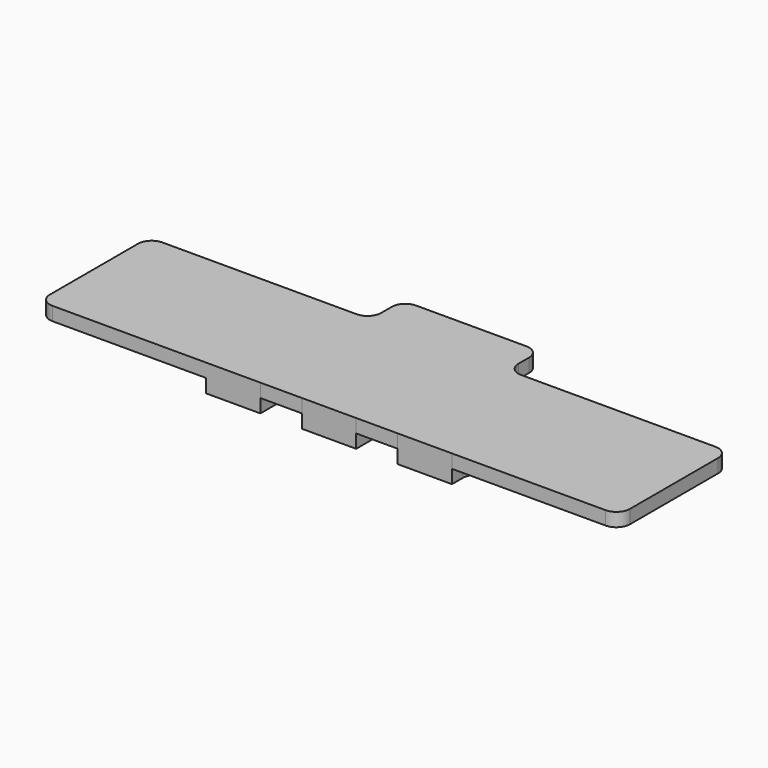
from build123d import *

# Parameters (mm, degrees)
F1_DEPTH = 0.75
F2_DEPTH = 0.75


# Not quite as in the source:
# - ends of sketch curves that miss each other by under 0.0002 mm in the source are joined


with BuildPart() as f1:
    # F0 (on Top) → F1 (new body)
    with BuildSketch(Plane.XY):
        with BuildLine():
            Line((-4.3542903055, 3.0103204122), (-15.1042902548, 3.0103204122))
            ThreePointArc((-15.1042902548, 3.0103204122), (-15.634620706, 2.7906503467), (-15.8542907714, 2.2603198956))
            Line((-15.8542907714, 2.2603198956), (-15.8542907714, -3.8396952234))
            ThreePointArc((-15.8542907714, -3.8396952234), (-15.634620706, -4.3700256746), (-15.1042902548, -4.58969574))
            Line((-15.1042902548, -4.58969574), (-6.6042903055, -4.58969574))
            Line((-6.6042903055, -4.58969574), (-6.6042903055, -3.8396876639))
            ThreePointArc((-6.6042903055, -3.8396876639), (-6.8239602196, -3.309357578), (-7.3542903055, -3.0896876639))
            Line((-7.3542903055, -3.0896876639), (-14.3542907714, -3.0896876639))
            Line((-14.3542907714, -3.0896876639), (-14.3542907714, 1.5103194803))
            Line((-14.3542907714, 1.5103194803), (-4.3542898395, 1.5103132679))
            ThreePointArc((-4.3542898395, 1.5103132679), (-3.8239600548, 1.2906431891), (-3.6042903055, 0.7603132679))
            Line((-3.6042903055, 0.7603132679), (-3.6042903055, -4.5896876639))
            Line((-3.6042903055, -4.5896876639), (-1.3042907714, -4.58969574))
            Line((-1.3042907714, -4.58969574), (-1.3042907714, -3.4706392285))
            ThreePointArc((-1.3042907714, -3.4706392285), (-1.3745455835, -3.153706188), (-1.5721480592, -2.8961492966))
            ThreePointArc((-1.5721480592, -2.8961492966), (-2.5098893785, -1.2818626098), (-2.2007190289, 0.5592495498))
            ThreePointArc((-2.2007190289, 0.5592495498), (-2.1287979009, 0.7369818479), (-2.1042903055, 0.9271417706))
            Line((-2.1042903055, 0.9271417706), (-2.1042903055, 3.7487632608))
            Line((-2.1042903055, 3.7487632608), (2.4957087627, 3.7487632608))
            Line((2.4957087627, 3.7487632608), (2.4957087627, 0.9271417706))
            ThreePointArc((2.4957087627, 0.9271417706), (2.5202163581, 0.7369818479), (2.5921374862, 0.5592495498))
            ThreePointArc((2.5921374862, 0.5592495498), (2.9013078357, -1.2818626098), (1.9635665164, -2.8961492966))
            ThreePointArc((1.9635665164, -2.8961492966), (1.7659640407, -3.153706188), (1.6957092286, -3.4706392285))
            Line((1.6957092286, -3.4706392285), (1.6957092286, -4.5896876639))
            Line((1.6957092286, -4.5896876639), (3.9957149822, -4.58969574))
            Line((3.9957149822, -4.58969574), (3.9957116586, 0.7603127188))
            ThreePointArc((3.9957116586, 0.7603127188), (4.2153814061, 1.290643318), (4.7457117418, 1.5103137014))
            Line((4.7457117418, 1.5103137014), (14.7457092286, 1.5103194803))
            Line((14.7457092286, 1.5103194803), (14.7457092286, -3.0896876639))
            Line((14.7457092286, -3.0896876639), (7.7457154989, -3.0896876639))
            ThreePointArc((7.7457154989, -3.0896876639), (7.2153850477, -3.3093577293), (6.9957149822, -3.8396881805))
            Line((6.9957149822, -3.8396881805), (6.9957149822, -4.5896876639))
            Line((6.9957149822, -4.5896876639), (15.495708712, -4.58969574))
            ThreePointArc((15.495708712, -4.58969574), (16.0260391632, -4.3700256746), (16.2457092286, -3.8396952234))
            Line((16.2457092286, -3.8396952234), (16.2457092286, 2.2603198956))
            ThreePointArc((16.2457092286, 2.2603198956), (16.0260391632, 2.7906503467), (15.495708712, 3.0103204122))
            Line((15.495708712, 3.0103204122), (4.7457149822, 3.0103204122))
            ThreePointArc((4.7457149822, 3.0103204122), (4.2153848964, 3.2299903263), (3.9957149822, 3.7603204122))
            Line((3.9957149822, 3.7603204122), (3.9957149822, 4.4987632608))
            ThreePointArc((3.9957149822, 4.4987632608), (3.7760450681, 5.0290933467), (3.2457149822, 5.2487632608))
            Line((3.2457149822, 5.2487632608), (-2.8542903055, 5.2487632608))
            ThreePointArc((-2.8542903055, 5.2487632608), (-3.3846203913, 5.0290933467), (-3.6042903055, 4.4987632608))
            Line((-3.6042903055, 4.4987632608), (-3.6042903055, 3.7603204122))
            ThreePointArc((-3.6042903055, 3.7603204122), (-3.8239602196, 3.2299903263), (-4.3542903055, 3.0103204122))
        make_face()
        with BuildLine():
            Line((-6.6042903055, -3.8396876639), (-6.6042903055, -4.58969574))
            Line((-6.6042903055, -4.58969574), (-3.6042903055, -4.58969574))
            Line((-3.6042903055, -4.58969574), (-3.6042903055, 0.7603132679))
            ThreePointArc((-3.6042903055, 0.7603132679), (-3.8239600548, 1.2906431891), (-4.3542898395, 1.5103132679))
            Line((-4.3542898395, 1.5103132679), (-14.3542907714, 1.5103194803))
            Line((-14.3542907714, 1.5103194803), (-14.3542907714, -3.0896876639))
            Line((-14.3542907714, -3.0896876639), (-7.3542903055, -3.0896876639))
            ThreePointArc((-7.3542903055, -3.0896876639), (-6.8239602196, -3.309357578), (-6.6042903055, -3.8396876639))
        make_face()
        with BuildLine():
            Line((3.9957116586, 0.7603127188), (3.9957149822, -4.5896876639))
            Line((3.9957149822, -4.5896876639), (6.9957149822, -4.58969574))
            Line((6.9957149822, -4.58969574), (6.9957149822, -3.8396881805))
            ThreePointArc((6.9957149822, -3.8396881805), (7.2153850477, -3.3093577293), (7.7457154989, -3.0896876639))
            Line((7.7457154989, -3.0896876639), (14.7457092286, -3.0896876639))
            Line((14.7457092286, -3.0896876639), (14.7457092286, 1.5103194803))
            Line((14.7457092286, 1.5103194803), (4.7457117418, 1.5103137014))
            ThreePointArc((4.7457117418, 1.5103137014), (4.2153814061, 1.290643318), (3.9957116586, 0.7603127188))
        make_face()
        with BuildLine():
            Line((-1.3042907714, -3.4706392285), (-1.3042907714, -4.5896876639))
            Line((-1.3042907714, -4.5896876639), (1.6957092286, -4.58969574))
            Line((1.6957092286, -4.58969574), (1.6957092286, -3.4706392285))
            ThreePointArc((1.6957092286, -3.4706392285), (1.7659640407, -3.153706188), (1.9635665164, -2.8961492966))
            ThreePointArc((1.9635665164, -2.8961492966), (2.9013078357, -1.2818626098), (2.5921374862, 0.5592495498))
            ThreePointArc((2.5921374862, 0.5592495498), (2.5202163581, 0.7369818479), (2.4957087627, 0.9271417706))
            Line((2.4957087627, 0.9271417706), (2.4957087627, 3.7487632608))
            Line((2.4957087627, 3.7487632608), (-2.1042903055, 3.7487632608))
            Line((-2.1042903055, 3.7487632608), (-2.1042903055, 0.9271417706))
            ThreePointArc((-2.1042903055, 0.9271417706), (-2.1287979009, 0.7369818479), (-2.2007190289, 0.5592495498))
            ThreePointArc((-2.2007190289, 0.5592495498), (-2.5098893785, -1.2818626098), (-1.5721480592, -2.8961492966))
            ThreePointArc((-1.5721480592, -2.8961492966), (-1.3745455835, -3.153706188), (-1.3042907714, -3.4706392285))
        make_face()
    extrude(amount=F1_DEPTH)

    # F0 (on Top) → F2 (join)
    with BuildSketch(Plane.XY):
        with BuildLine():
            Line((-6.6042903055, -3.8396876639), (-6.6042903055, -4.58969574))
            Line((-6.6042903055, -4.58969574), (-3.6042903055, -4.58969574))
            Line((-3.6042903055, -4.58969574), (-3.6042903055, 0.7603132679))
            ThreePointArc((-3.6042903055, 0.7603132679), (-3.8239600548, 1.2906431891), (-4.3542898395, 1.5103132679))
            Line((-4.3542898395, 1.5103132679), (-14.3542907714, 1.5103194803))
            Line((-14.3542907714, 1.5103194803), (-14.3542907714, -3.0896876639))
            Line((-14.3542907714, -3.0896876639), (-7.3542903055, -3.0896876639))
            ThreePointArc((-7.3542903055, -3.0896876639), (-6.8239602196, -3.309357578), (-6.6042903055, -3.8396876639))
        make_face()
        with BuildLine():
            Line((-1.3042907714, -3.4706392285), (-1.3042907714, -4.5896876639))
            Line((-1.3042907714, -4.5896876639), (1.6957092286, -4.58969574))
            Line((1.6957092286, -4.58969574), (1.6957092286, -3.4706392285))
            ThreePointArc((1.6957092286, -3.4706392285), (1.7659640407, -3.153706188), (1.9635665164, -2.8961492966))
            ThreePointArc((1.9635665164, -2.8961492966), (2.9013078357, -1.2818626098), (2.5921374862, 0.5592495498))
            ThreePointArc((2.5921374862, 0.5592495498), (2.5202163581, 0.7369818479), (2.4957087627, 0.9271417706))
            Line((2.4957087627, 0.9271417706), (2.4957087627, 3.7487632608))
            Line((2.4957087627, 3.7487632608), (-2.1042903055, 3.7487632608))
            Line((-2.1042903055, 3.7487632608), (-2.1042903055, 0.9271417706))
            ThreePointArc((-2.1042903055, 0.9271417706), (-2.1287979009, 0.7369818479), (-2.2007190289, 0.5592495498))
            ThreePointArc((-2.2007190289, 0.5592495498), (-2.5098893785, -1.2818626098), (-1.5721480592, -2.8961492966))
            ThreePointArc((-1.5721480592, -2.8961492966), (-1.3745455835, -3.153706188), (-1.3042907714, -3.4706392285))
        make_face()
        with BuildLine():
            Line((3.9957116586, 0.7603127188), (3.9957149822, -4.5896876639))
            Line((3.9957149822, -4.5896876639), (6.9957149822, -4.58969574))
            Line((6.9957149822, -4.58969574), (6.9957149822, -3.8396881805))
            ThreePointArc((6.9957149822, -3.8396881805), (7.2153850477, -3.3093577293), (7.7457154989, -3.0896876639))
            Line((7.7457154989, -3.0896876639), (14.7457092286, -3.0896876639))
            Line((14.7457092286, -3.0896876639), (14.7457092286, 1.5103194803))
            Line((14.7457092286, 1.5103194803), (4.7457117418, 1.5103137014))
            ThreePointArc((4.7457117418, 1.5103137014), (4.2153814061, 1.290643318), (3.9957116586, 0.7603127188))
        make_face()
    extrude(amount=-F2_DEPTH)


solid = f1.part
